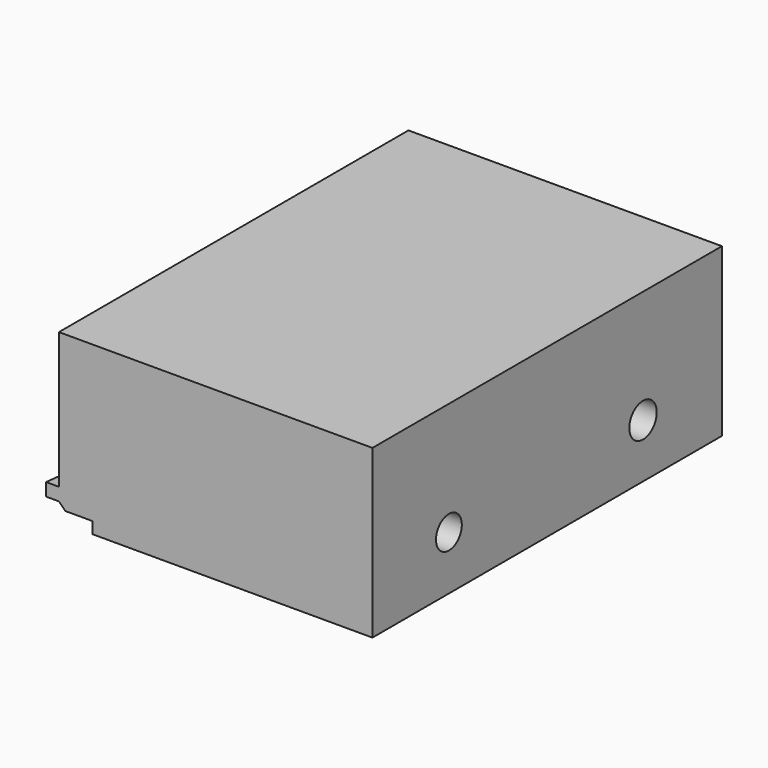
from build123d import *

# Parameters (mm, degrees)
F0_W     = 77.47
F0_H     = 107.95
F1_DEPTH = 41.275
F2_R     = 3.9878
F2_R_2   = 4.2274185689
F3_DEPTH = 77.471
F5_DEPTH = 107.951
F7_DEPTH = 3.175


# Not quite as in the source:
# - a pattern or mirror of a feature is missing from the dataset's text; its kind, count and spacing are read off the source's solid


with BuildPart() as f1:
    # F0 (on Top) → F1 (new body)
    with BuildSketch(Plane.XY):
        Rectangle(F0_W, F0_H)
    extrude(amount=F1_DEPTH)

    # F2 (on face) → F3 (cut, through all)
    with BuildSketch(Plane.YZ.offset(38.735)):
        with Locations((-30.3550828248, 13.335)):
            Circle(F2_R)
        with Locations((29.6055749059, 13.335)):
            Circle(F2_R_2)
    extrude(amount=-F3_DEPTH, mode=Mode.SUBTRACT)

    # F4 (on face) → F5 (cut, through all)
    with BuildSketch(Plane(origin=(0, 53.975, 0), x_dir=(-1, 0, 0), z_dir=(0, 1, 0))):
        Polygon((38.735, 0), (38.735, 4.445), (37.1475, 2.8575), (30.48, 2.8575), (30.48, 0), align=None)
    extrude(amount=-F5_DEPTH, mode=Mode.SUBTRACT)

    # F6 (on face) → F7 (join)
    with BuildSketch(Plane(origin=(-38.735, 0, 0), x_dir=(0, -1, 0), z_dir=(-1, 0, 0))):
        Polygon((-53.975, 7.62), (-53.975, 4.445), (-43.815, 4.445), (-43.815, 6.7311151786), align=None)
    f7 = extrude(amount=F7_DEPTH)

    # F7_copies: F7 across plane
    add(f7.mirror(Plane(origin=(0, 0, 0), x_dir=(0, 0, -1), z_dir=(0, -1, 0))))


solid = f1.part
